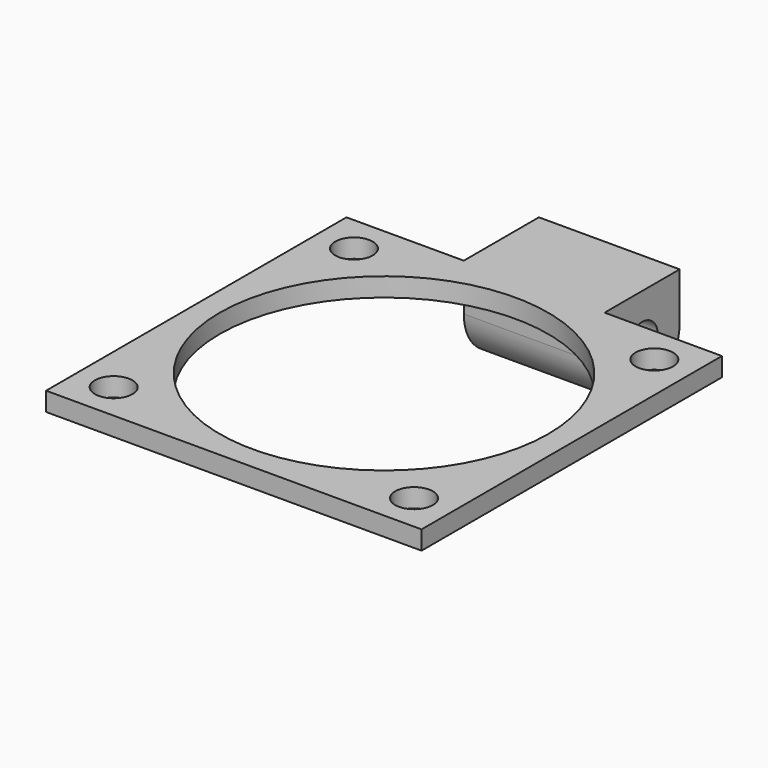
from build123d import *

# Parameters (mm, degrees)
F0_W     = 15
F0_H     = 10
F1_DEPTH = 2
F2_R     = 2
F3_DEPTH = 2.001
F4_R     = 17.5
F5_DEPTH = 2.001
F6_W     = 15
F6_H     = 10
F7_DEPTH = 8
F8_R     = 2.1
F9_DEPTH = 27.501
F10_R    = 4.99999


# Not quite as in the source:
# - a fillet or chamfer is up to 0.001 mm smaller than in the source, because OpenCascade refuses the exact size


with BuildPart() as f1:
    # F0 (on Top) → F1 (new body)
    with BuildSketch(Plane.XY):
        Polygon((0, 40), (0, 0), (40, 0), (40, 40), (27.5, 40), (12.5, 40), align=None)
        with Locations((20, 45)):
            Rectangle(F0_W, F0_H)
    extrude(amount=F1_DEPTH)

    # F2 (on face) → F3 (cut, through all)
    with BuildSketch(Plane.XY.offset(2)):
        with Locations((4, 36)):
            Circle(F2_R)
        with Locations((36, 36)):
            Circle(F2_R)
        with Locations((4, 4)):
            Circle(F2_R)
        with Locations((36, 4)):
            Circle(F2_R)
    extrude(amount=-F3_DEPTH, mode=Mode.SUBTRACT)

    # F4 (on face) → F5 (cut, through all)
    with BuildSketch(Plane.XY.offset(2)):
        with Locations((20, 20)):
            Circle(F4_R)
    extrude(amount=-F5_DEPTH, mode=Mode.SUBTRACT)

    # F6 (on face) → F7 (join)
    with BuildSketch(Plane(origin=(0, 0, 0), x_dir=(1, 0, 0), z_dir=(0, 0, -1))):
        with Locations((20, -45)):
            Rectangle(F6_W, F6_H)
    extrude(amount=F7_DEPTH)

    # F8 (on face) → F9 (cut, through all)
    with BuildSketch(Plane.YZ.offset(27.5)):
        with Locations((45, -3)):
            Circle(F8_R)
    extrude(amount=-F9_DEPTH, mode=Mode.SUBTRACT)

    # F10 (radius 5 in the source; OpenCascade refuses exactly that, so slightly less here)
    f10_edges = [f1.edges().sort_by_distance(p)[0] for p in [
        (20, 50, -8),
        (20, 40, -8),
    ]]
    fillet(f10_edges, radius=F10_R)


solid = f1.part
